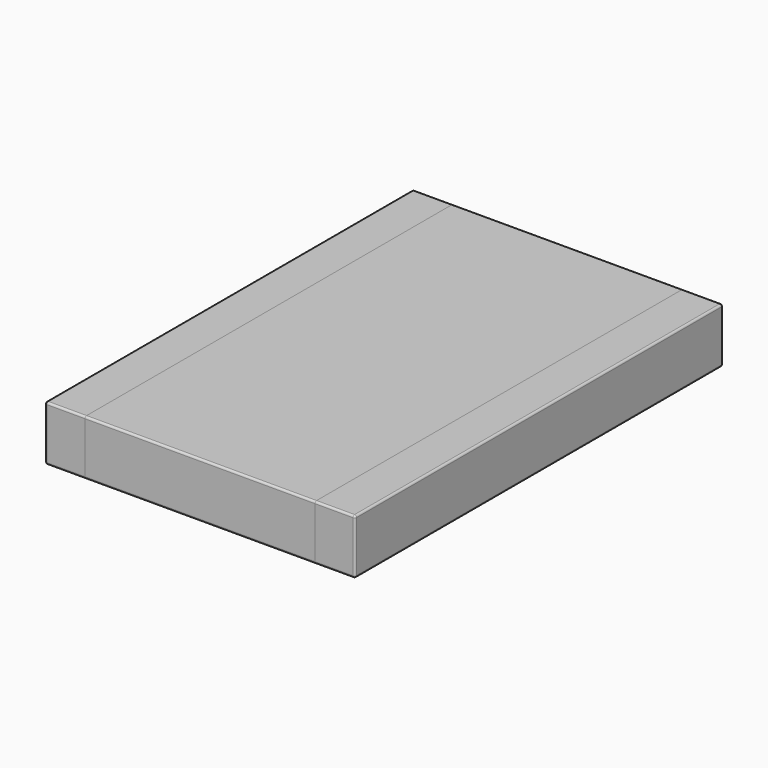
from build123d import *

# Parameters (mm, degrees)
F2_W     = 2.3
F2_H     = 4.6
F3_DEPTH = 0.53
F2_W_2   = 0.4
F4_DEPTH = 0.55
F5_DEPTH = 0.55
F6_DEPTH = 0.02
F7_R     = 0.01999
F7_2_R   = 0.01999
F7_3_R   = 0.01999
F7_4_R   = 0.01999


# Not quite as in the source:
# - a fillet or chamfer is up to 0.001 mm smaller than in the source, because OpenCascade refuses the exact size


with BuildPart() as f3:
    # F2 (on Top) → F3 (new body)
    with BuildSketch(Plane.XY):
        Rectangle(F2_W, F2_H)
    extrude(amount=F3_DEPTH)


with BuildPart() as f4:
    # F2 (on Top) → F4 (new body)
    with BuildSketch(Plane.XY):
        with Locations((-1.35, 0)):
            Rectangle(F2_W_2, F2_H)
    extrude(amount=F4_DEPTH)

    # F7 (radius 0.02 in the source; OpenCascade refuses exactly that, so slightly less here)
    f7_edges = [f4.edges().sort_by_distance(p)[0] for p in [
        (-1.35, -2.3, 0.55),
        (-1.55, 2.3, 0.275),
        (-1.55, -2.3, 0.275),
        (-1.55, 0, 0),
        (-1.55, 0, 0.55),
        (-1.35, 2.3, 0.55),
        (-1.35, 2.3, 0),
        (-1.35, -2.3, 0),
    ]]
    fillet(f7_edges, radius=F7_R)


with BuildPart() as f5:
    # F2 (on Top) → F5 (new body)
    with BuildSketch(Plane.XY):
        with Locations((1.35, 0)):
            Rectangle(F2_W_2, F2_H)
    extrude(amount=F5_DEPTH)

    # F7#2 (radius 0.02 in the source; OpenCascade refuses exactly that, so slightly less here)
    f7_2_edges = [f5.edges().sort_by_distance(p)[0] for p in [
        (1.35, -2.3, 0.55),
        (1.55, -2.3, 0.275),
        (1.55, 2.3, 0.275),
        (1.55, 0, 0),
        (1.55, 0, 0.55),
        (1.35, 2.3, 0.55),
        (1.35, 2.3, 0),
        (1.35, -2.3, 0),
    ]]
    fillet(f7_2_edges, radius=F7_2_R)


with BuildPart() as f6:
    # F6 (new): a face of the model
    f6_faces = [f3.part.faces().sort_by_distance(p)[0] for p in [
        (0, 0, 0.53),
    ]]
    extrude(f6_faces, amount=F6_DEPTH)

    # F7#4 (radius 0.02 in the source; OpenCascade refuses exactly that, so slightly less here)
    f7_4_edges = [f6.edges().sort_by_distance(p)[0] for p in [
        (0, -2.3, 0.55),
        (0, 2.3, 0.55),
    ]]
    fillet(f7_4_edges, radius=F7_4_R)


with BuildPart() as f3_1:
    add(f3.part)

    # F7#3 (radius 0.02 in the source; OpenCascade refuses exactly that, so slightly less here)
    f7_3_edges = [f3_1.edges().sort_by_distance(p)[0] for p in [
        (0, 2.3, 0),
        (0, -2.3, 0),
    ]]
    fillet(f7_3_edges, radius=F7_3_R)


solid = Compound([f4.part, f5.part, f6.part, f3_1.part])
